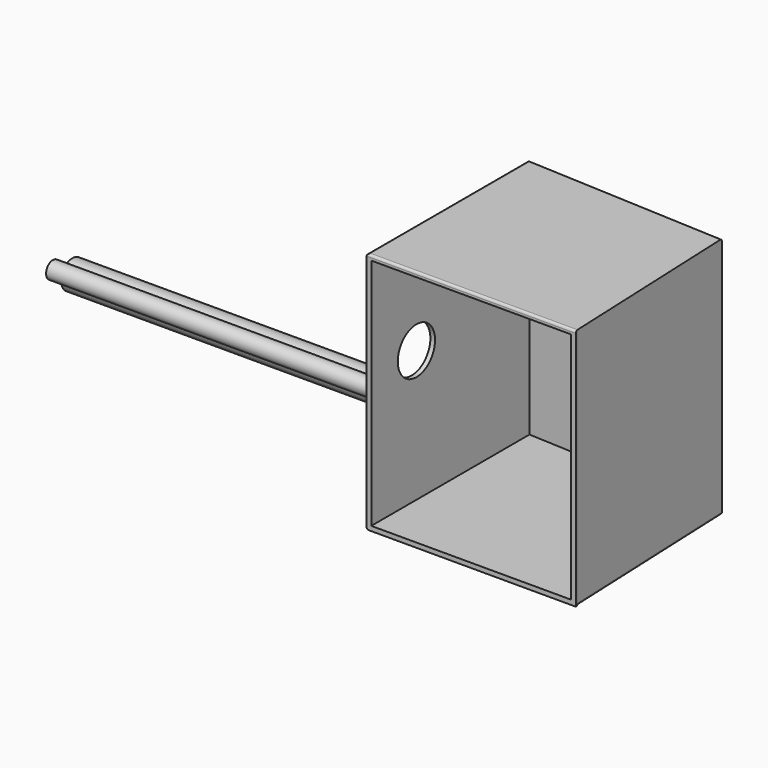
from build123d import *

# Parameters (mm, degrees)
F1_DEPTH  = 132.334
F2_T      = -2.54
F3_DEPTH  = 0.762
F5_D      = 25.4
F5_DEPTH  = 5.08
F5_TIP    = 7.6309298617
F9_R      = 1.2264204897
F7_R      = 7.7162508116
F7_R_2    = 4.6438728955
F10_DEPTH = 189.738


with BuildPart() as f1:
    # F0 (on Top) → F1 (new body)
    with BuildSketch(Plane.XY):
        Polygon((52.318636328, 57.9638108611), (-57.1821704507, 63.2404088974), (-57.1821704507, -47.161385417), (56.8056404591, -47.161385417), align=None)
    extrude(amount=F1_DEPTH)

    # F2
    f2_openings = [f1.faces().sort_by_distance(p)[0] for p in [
        (-0.188265, -47.161385, 66.167),
    ]]
    offset(amount=F2_T, openings=f2_openings)

    # F3 (add): a face of the model
    f3_faces = [f1.faces().sort_by_distance(p)[0] for p in [
        (-55.4355878276, -47.161385417, 66.167),
    ]]
    extrude(f3_faces, amount=-F3_DEPTH)

    # F5 (one way)
    with BuildSketch(Plane.YZ.offset(-54.6421704507)):
        with Locations((-16.4339449257, 74.0607306361)):
            Circle(F5_D / 2)
    extrude(amount=-F5_DEPTH, mode=Mode.SUBTRACT)
    with Locations(Plane.YZ.offset(-54.6421704507)):
        with Locations((-16.4339449257, 74.0607306361)):
            with Locations((0, 0, -(F5_DEPTH + F5_TIP / 2))):  # 118° drill point
                Cone(0, F5_D / 2, F5_TIP, mode=Mode.SUBTRACT)

    # F9
    f9_edges = [f1.edges().sort_by_distance(p)[0] for p in [
        (-57.18217, 8.039512, 132.334),
        (-2.431767, 60.60211, 132.334),
        (-0.188265, -47.161385, 132.334),
        (-57.18217, 8.039512, 0),
        (54.545876, 5.782213, 0),
        (-2.431767, 60.60211, 0),
    ]]
    fillet(f9_edges, radius=F9_R)

    # F7 (on face) → F10 (join)
    with BuildSketch(Plane.YZ.offset(-54.6421704507)):
        with Locations((-13.5401813313, 47.8832386434)):
            Circle(F7_R)
        with Locations((-26.8557239324, 55.4966442287)):
            Circle(F7_R_2)
    extrude(amount=-F10_DEPTH)


solid = f1.part
